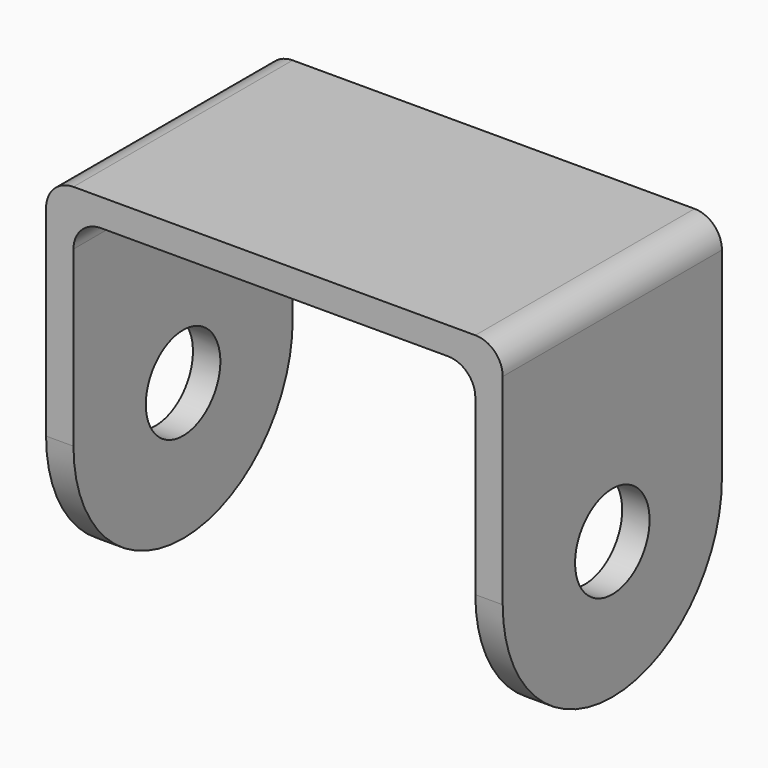
from build123d import *

# Parameters (mm, degrees)
F1_DEPTH = 30
F2_R     = 5.1
F3_DEPTH = 50.0010000522
F4_R     = 14.99999
F5_R     = 3


# Not quite as in the source:
# - a fillet or chamfer is up to 0.001 mm smaller than in the source, because OpenCascade refuses the exact size


with BuildPart() as f1:
    # F0 (on Front) → F1 (new body)
    with BuildSketch(Plane.XZ):
        Polygon((-3.0000000261, 0), (0, 0), (0, 37), (44, 37), (44, 0), (47.0000000261, 0), (47.0000000261, 40.0000000261), (-3.0000000261, 40.0000000261), align=None)
    extrude(amount=F1_DEPTH)

    # F2 (on face) → F3 (cut, through all)
    with BuildSketch(Plane(origin=(-3.0000000261, 0, 0), x_dir=(0, -1, 0), z_dir=(-1, 0, 0))):
        with Locations((15, 15.0000000261)):
            Circle(F2_R)
    extrude(amount=-F3_DEPTH, mode=Mode.SUBTRACT)

    # F4 (radius 15 in the source; OpenCascade refuses exactly that, so slightly less here)
    f4_edges = [f1.edges().sort_by_distance(p)[0] for p in [
        (45.5, 0, 0),
        (45.5, -30, 0),
        (-1.5, -30, 0),
        (-1.5, 0, 0),
    ]]
    fillet(f4_edges, radius=F4_R)

    # F5
    f5_edges = [f1.edges().sort_by_distance(p)[0] for p in [
        (0, -15, 37),
        (44, -15, 37),
        (47, -15, 40),
        (-3, -15, 40),
    ]]
    fillet(f5_edges, radius=F5_R)


solid = f1.part
